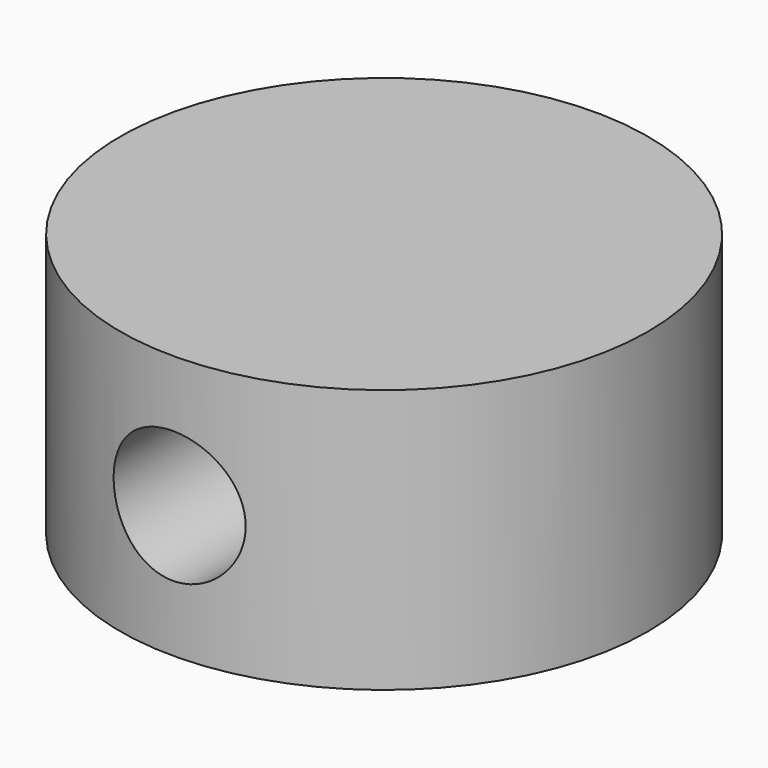
from build123d import *

# Parameters (mm, degrees)
F2_R     = 3
F3_DEPTH = 3
F4_R     = 0.75
F5_DEPTH = 3.31


# Not quite as in the source:
# - a feature names something its author has since deleted; it is built from what else it names
# - the program builds the solid bodies; features that only make, move or delete a surface that nothing else refers to are left out


with BuildPart() as f3:
    # F2 (on Top) → F3 (new body)
    with BuildSketch(Plane.XY):
        with Locations((-39.4553284803, 0)):
            Circle(F2_R)
    extrude(amount=F3_DEPTH)

    # F4 (on Front) → F5 (cut, symmetric)
    with BuildSketch(Plane.XZ):
        with Locations((-39.4553284803, 1.5)):
            Circle(F4_R)
    extrude(amount=F5_DEPTH, both=True, mode=Mode.SUBTRACT)


with BuildPart() as f3_1:
    # F8: moved
    add(f3.part.moved(Location((0.033225133, 0, -0.5896431374))))


solid = f3_1.part
